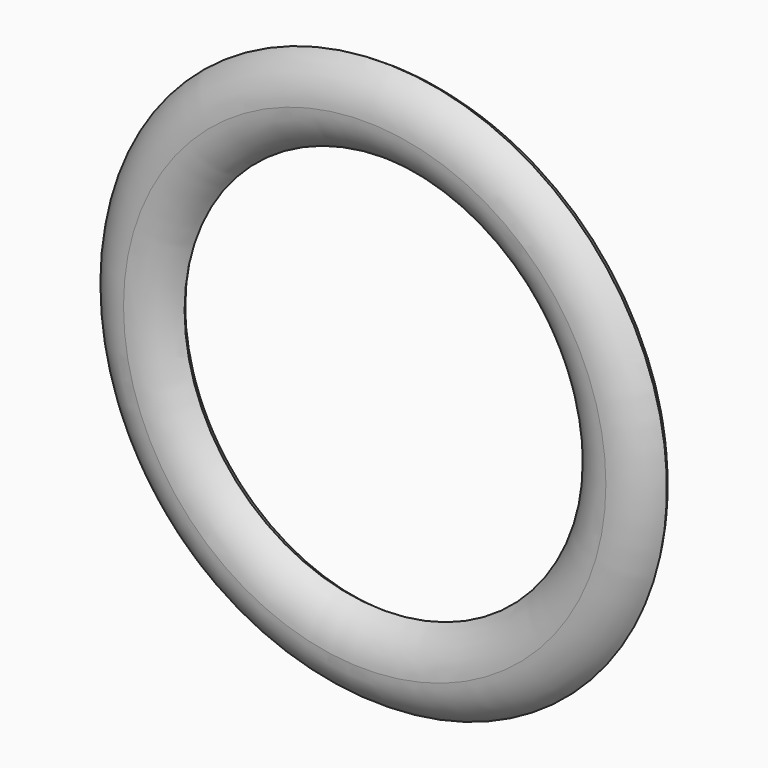
from build123d import *

# Parameters (mm, degrees)
F0_W = 12.7
F0_H = 6.35
F2_R = 6.34999
F3_R = 6.34999


# Not quite as in the source:
# - a fillet or chamfer is up to 0.001 mm smaller than in the source, because OpenCascade refuses the exact size


with BuildPart() as f1:
    # F0 (on Top) → F1 (revolve)
    with BuildSketch(Plane.XY):
        Rectangle(F0_W, F0_H)
    revolve(axis=Axis((31.75, -0.4141320733, 0), (0, -1, 0)))

    # F2 (radius 6.35 in the source; OpenCascade refuses exactly that, so slightly less here)
    f2_edges = [f1.edges().sort_by_distance(p)[0] for p in [
        (57.15, 3.175, 0),
    ]]
    fillet(f2_edges, radius=F2_R)

    # F3 (radius 6.35 in the source; OpenCascade refuses exactly that, so slightly less here)
    f3_edges = [f1.edges().sort_by_distance(p)[0] for p in [
        (69.85, 3.175, 0),
    ]]
    fillet(f3_edges, radius=F3_R)

    # F4: F1 across plane


with BuildPart() as f1_1:
    add(f1.part)
    add(f1.part.mirror(Plane.XZ), mode=Mode.INTERSECT)


solid = f1_1.part
